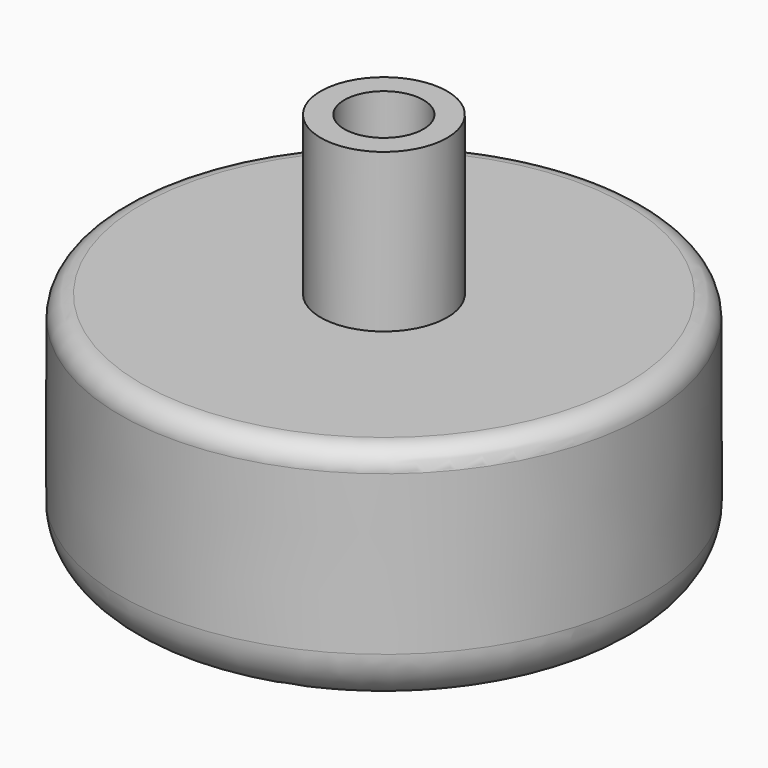
from build123d import *


# Not quite as in the source:
# - a feature names something its author has since deleted; it is built from what else it names


with BuildPart() as f1:
    # F0 (on Front) → F1 (revolve)
    with BuildSketch(Plane.XZ):
        with BuildLine():
            Line((0, 47.625), (0, 21.59))
            Line((0, 21.59), (1.6002, 21.59))
            Line((1.6002, 21.59), (1.6002, 0.6053799298))
            Line((1.6002, 0.6053799298), (27.7014960486, 10.4798960957))
            ThreePointArc((27.7014960486, 10.4798960957), (30.6836253917, 12.8163260486), (31.8045894836, 16.435088247))
            Line((31.8045894836, 16.435088247), (31.7563839592, 35.5664000652))
            ThreePointArc((31.7563839592, 35.5664000652), (31.0101790546, 37.3583125654), (29.2163920223, 38.1))
            Line((29.2163920223, 38.1), (7.62, 38.1))
            Line((7.62, 38.1), (7.62, 57.15))
            Line((7.62, 57.15), (4.7625, 57.15))
            Line((4.7625, 57.15), (4.7625, 47.625))
            Line((4.7625, 47.625), (0, 47.625))
        make_face()
    revolve(axis=Axis((0, 0, 28.575), (0, 0, 1)))


solid = f1.part
